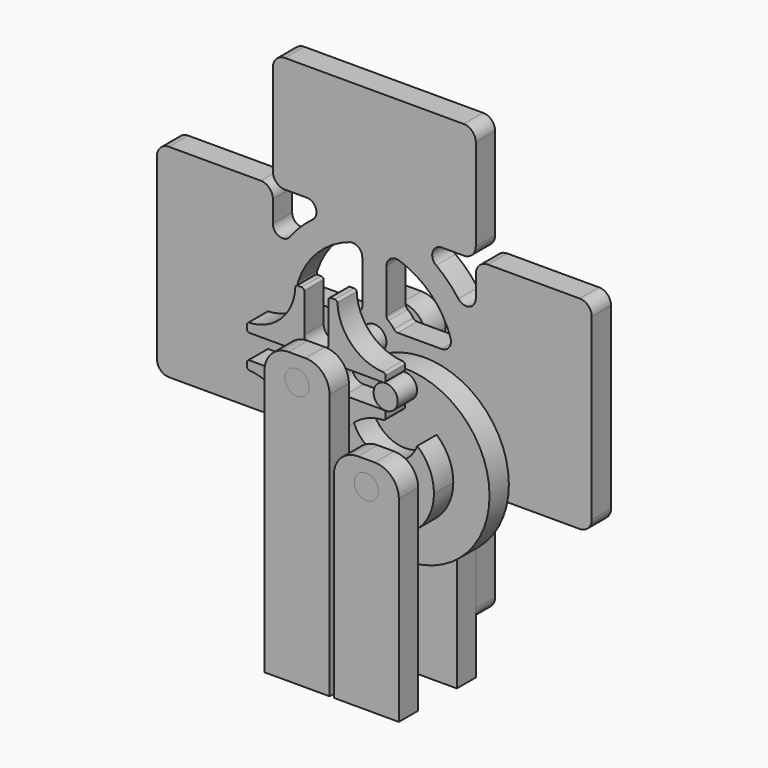
from build123d import *

# Parameters (mm, degrees)
F0_R          = 22.225
F0_R_2        = 3.175
F1_DEPTH      = 6.35
F2_DEPTH      = 6.35
F3_R          = 3.175
F4_DEPTH      = 6.35
F5_DEPTH      = 12.7
F5_DEPTH_BACK = 12.7
F6_DEPTH      = 12.7
F6_DEPTH_BACK = 25.4
F7_R          = 3.17499
F8_R          = 0.635
F9_W          = 17.0939071104
F9_H          = 57.9826636136
F9_R          = 3.175
F10_DEPTH     = 6.35
F9_H_2        = 76.2
F11_W         = 17.0939071104
F11_H         = 57.9826636136
F11_R         = 3.175
F12_DEPTH     = 6.35
F13_R         = 3.175
F13_W         = 11.8072872561
F13_H         = 12.7
F13_W_2       = 12.7
F13_H_2       = 11.8072872561
F14_DEPTH     = 6.35
F16_DEPTH     = 6.35
F17_R         = 2.54
F18_R         = 1.27
F19_W         = 17.0939071104
F19_H         = 76.2
F19_R         = 3.175
F20_DEPTH     = 6.35
F21_R         = 6.35
F21_2_R       = 6.35
F21_3_R       = 6.35
F21_4_R       = 6.35


# Not quite as in the source:
# - a fillet or chamfer is up to 0.001 mm smaller than in the source, because OpenCascade refuses the exact size
# - a feature names something its author has since deleted; it is built from what else it names


with BuildPart() as f1:
    # F0 (on Front) → F1 (new body)
    with BuildSketch(Plane.XZ):
        Circle(F0_R)
        with BuildLine():
            ThreePointArc((8.3277048309, 9.5885), (11.5553418676, 5.2691625828), (12.7, 0))
            ThreePointArc((12.7, 0), (-5.2691625828, -11.5553418676), (-8.3277048309, 9.5885))
            ThreePointArc((-8.3277048309, 9.5885), (0, 12.7), (8.3277048309, 9.5885))
        make_face(mode=Mode.SUBTRACT)
        with Locations((0, 18.2173363864)):
            Circle(F0_R_2, mode=Mode.SUBTRACT)
        with Locations((0, 18.2173363864)):
            Circle(F0_R_2)
        with BuildLine():
            ThreePointArc((-8.3277048309, 9.5885), (0, 3.81), (8.3277048309, 9.5885))
            ThreePointArc((8.3277048309, 9.5885), (0, 12.7), (-8.3277048309, 9.5885))
        make_face()
        with BuildLine():
            ThreePointArc((-8.3277048309, 9.5885), (-5.2691625828, -11.5553418676), (12.7, 0))
            ThreePointArc((12.7, 0), (11.5553418676, 5.2691625828), (8.3277048309, 9.5885))
            ThreePointArc((8.3277048309, 9.5885), (0, 3.81), (-8.3277048309, 9.5885))
        make_face()
        Circle(F0_R_2, mode=Mode.SUBTRACT)
    extrude(amount=-F1_DEPTH)

    # F0 (on Front) → F2 (join)
    with BuildSketch(Plane.XZ):
        with Locations((0, 18.2173363864)):
            Circle(F0_R_2)
        with BuildLine():
            ThreePointArc((-8.3277048309, 9.5885), (-5.2691625828, -11.5553418676), (12.7, 0))
            ThreePointArc((12.7, 0), (11.5553418676, 5.2691625828), (8.3277048309, 9.5885))
            ThreePointArc((8.3277048309, 9.5885), (0, 3.81), (-8.3277048309, 9.5885))
        make_face()
        Circle(F0_R_2, mode=Mode.SUBTRACT)
    extrude(amount=F2_DEPTH)


with BuildPart() as f4:
    # F3 (on face) → F4 (new body)
    with BuildSketch(Plane.XZ):
        with BuildLine():
            Line((-15.0423363864, 0), (-12.7, 0))
            ThreePointArc((-12.7, 0), (-11.5553418676, 5.2691625828), (-8.3277048309, 9.5885))
            ThreePointArc((-8.3277048309, 9.5885), (-4.445, 11.8967211869), (0, 12.7))
            Line((0, 12.7), (0, 15.0423363864))
            Line((0, 15.0423363864), (-13.97, 15.0423363864))
            Line((-13.97, 15.0423363864), (-13.97, 17.2855351378))
            ThreePointArc((-13.97, 17.2855351378), (-15.7154482119, 15.7154482119), (-17.2855351378, 13.97))
            Line((-17.2855351378, 13.97), (-15.0423363864, 13.97))
            Line((-15.0423363864, 13.97), (-15.0423363864, 0))
        make_face()
        with BuildLine():
            Line((-23.7346727729, 0), (-22.225, 0))
            ThreePointArc((-22.225, 0), (-22.0158499857, 3.0418702151), (-21.3923363864, 6.0264889388))
            Line((-21.3923363864, 6.0264889388), (-21.3923363864, 13.97))
            Line((-21.3923363864, 13.97), (-17.2855351378, 13.97))
            ThreePointArc((-17.2855351378, 13.97), (-15.7154482119, 15.7154482119), (-13.97, 17.2855351378))
            Line((-13.97, 17.2855351378), (-13.97, 21.3923363864))
            Line((-13.97, 21.3923363864), (-6.0264889388, 21.3923363864))
            ThreePointArc((-6.0264889388, 21.3923363864), (-3.0418702151, 22.0158499857), (0, 22.225))
            Line((0, 22.225), (0, 23.7346727729))
            ThreePointArc((0, 23.7346727729), (-8.9802561211, 27.4544166518), (-12.7, 36.4346727729))
            Line((-12.7, 36.4346727729), (-15.0423363864, 36.4346727729))
            Line((-15.0423363864, 36.4346727729), (-15.0423363864, 22.4646727729))
            Line((-15.0423363864, 22.4646727729), (-21.3923363864, 22.4646727729))
            Line((-21.3923363864, 22.4646727729), (-21.3923363864, 36.4346727729))
            Line((-21.3923363864, 36.4346727729), (-23.7346727729, 36.4346727729))
            ThreePointArc((-23.7346727729, 36.4346727729), (-27.4544166518, 27.4544166518), (-36.4346727729, 23.7346727729))
            Line((-36.4346727729, 23.7346727729), (-36.4346727729, 21.3923363864))
            Line((-36.4346727729, 21.3923363864), (-22.4646727729, 21.3923363864))
            Line((-22.4646727729, 21.3923363864), (-22.4646727729, 15.0423363864))
            Line((-22.4646727729, 15.0423363864), (-36.4346727729, 15.0423363864))
            Line((-36.4346727729, 15.0423363864), (-36.4346727729, 12.7))
            ThreePointArc((-36.4346727729, 12.7), (-27.4544166518, 8.9802561211), (-23.7346727729, 0))
        make_face()
        with Locations((-18.2173363864, 18.2173363864)):
            Circle(F3_R, mode=Mode.SUBTRACT)
        with BuildLine():
            Line((-6.0264889388, 21.3923363864), (0, 21.3923363864))
            Line((0, 21.3923363864), (0, 22.225))
            ThreePointArc((0, 22.225), (-3.0418702151, 22.0158499857), (-6.0264889388, 21.3923363864))
        make_face()
        with BuildLine():
            Line((-22.225, 0), (-21.3923363864, 0))
            Line((-21.3923363864, 0), (-21.3923363864, 6.0264889388))
            ThreePointArc((-21.3923363864, 6.0264889388), (-22.0158499857, 3.0418702151), (-22.225, 0))
        make_face()
    extrude(amount=F4_DEPTH)

    # F7 (radius 3.175 in the source; OpenCascade refuses exactly that, so slightly less here)
    f7_edges = [f4.edges().sort_by_distance(p)[0] for p in [
        (-15.042336, -3.175, 22.464673),
        (-21.392336, -3.175, 22.464673),
        (-13.97, -3.175, 21.392336),
        (-13.97, -3.175, 15.042336),
        (-15.042336, -3.175, 13.97),
        (-21.392336, -3.175, 13.97),
        (-22.464673, -3.175, 15.042336),
        (-22.464673, -3.175, 21.392336),
    ]]
    fillet(f7_edges, radius=F7_R)

    # F8
    f8_edges = [f4.edges().sort_by_distance(p)[0] for p in [
        (-12.7, -3.175, 36.434673),
        (-15.042336, -3.175, 36.434673),
        (-21.392336, -3.175, 36.434673),
        (-23.734673, -3.175, 36.434673),
        (-36.434673, -3.175, 23.734673),
        (0, -3.175, 23.734673),
        (0, -3.175, 21.392336),
        (0, -3.175, 12.7),
        (-36.434673, -3.175, 15.042336),
        (-21.392336, -3.175, 0),
        (-36.434673, -3.175, 21.392336),
        (-36.434673, -3.175, 12.7),
        (-23.734673, -3.175, 0),
        (-15.042336, -3.175, 0),
        (-12.7, -3.175, 0),
        (0, -3.175, 15.042336),
    ]]
    fillet(f8_edges, radius=F8_R)


with BuildPart() as f5:
    # F0 (on Front) → F5 (new body, two sides)
    with BuildSketch(Plane.XZ) as f5_sk:
        Circle(F0_R_2)
    extrude(amount=F5_DEPTH)
    extrude(f5_sk.sketch, amount=-F5_DEPTH_BACK)


with BuildPart() as f6:
    # F3 (on face) → F6 (new body, two sides)
    with BuildSketch(Plane.XZ) as f6_sk:
        with Locations((-18.2173363864, 18.2173363864)):
            Circle(F3_R)
    extrude(amount=F6_DEPTH)
    extrude(f6_sk.sketch, amount=-F6_DEPTH_BACK)


with BuildPart() as f10:
    # F9 (on face) → F10 (new body)
    with BuildSketch(Plane.XZ.offset(6.35)):
        with Locations((0, -22.6413318068)):
            Rectangle(F9_W, F9_H)
        Circle(F9_R, mode=Mode.SUBTRACT)
    extrude(amount=F10_DEPTH)

    # F21
    f21_edges = [f10.edges().sort_by_distance(p)[0] for p in [
        (8.546954, -9.525, 6.35),
        (-8.546954, -9.525, 6.35),
    ]]
    fillet(f21_edges, radius=F21_R)


with BuildPart() as f10b:
    # F9 (on face) → F10, piece 2 (new body)
    with BuildSketch(Plane.XZ.offset(6.35)):
        with Locations((-18.2173363864, -13.5326636136)):
            Rectangle(F9_W, F9_H_2)
        with Locations((-18.2173363864, 18.2173363864)):
            Circle(F9_R, mode=Mode.SUBTRACT)
    extrude(amount=F10_DEPTH)

    # F21#3
    f21_3_edges = [f10b.edges().sort_by_distance(p)[0] for p in [
        (-9.670383, -9.525, 24.567336),
        (-26.76429, -9.525, 24.567336),
    ]]
    fillet(f21_3_edges, radius=F21_3_R)


with BuildPart() as f12:
    # F11 (on face) → F12 (new body)
    with BuildSketch(Plane(origin=(0, 6.35, 0), x_dir=(-1, 0, 0), z_dir=(0, 1, 0))):
        with Locations((0, -22.6413318068)):
            Rectangle(F11_W, F11_H)
        Circle(F11_R, mode=Mode.SUBTRACT)
    extrude(amount=F12_DEPTH)

    # F21#2
    f21_2_edges = [f12.edges().sort_by_distance(p)[0] for p in [
        (8.546954, 9.525, 6.35),
        (-8.546954, 9.525, 6.35),
    ]]
    fillet(f21_2_edges, radius=F21_2_R)


with BuildPart() as f14:
    # F13 (on face) → F14 (new body)
    with BuildSketch(Plane(origin=(0, 12.7, 0), x_dir=(-1, 0, 0), z_dir=(0, 1, 0))):
        with BuildLine():
            ThreePointArc((44.8873363864, 11.8673363864), (45.4458475553, 15.0205286778), (45.6328684805, 18.2173363864))
            ThreePointArc((45.6328684805, 18.2173363864), (45.4458475553, 21.4141440951), (44.8873363864, 24.5673363864))
            Line((44.8873363864, 24.5673363864), (44.8873363864, 11.8673363864))
        make_face()
        with BuildLine():
            ThreePointArc((44.8873363864, 24.5673363864), (45.4458475553, 21.4141440951), (45.6328684805, 18.2173363864))
            ThreePointArc((45.6328684805, 18.2173363864), (45.4458475553, 15.0205286778), (44.8873363864, 11.8673363864))
            Line((44.8873363864, 11.8673363864), (44.8873363864, -5.2776636136))
            ThreePointArc((44.8873363864, -5.2776636136), (45.8172723562, -7.5227276438), (48.0623363864, -8.4526636136))
            Line((48.0623363864, -8.4526636136), (72.1923363864, -8.4526636136))
            ThreePointArc((72.1923363864, -8.4526636136), (74.4374004167, -7.5227276438), (75.3673363864, -5.2776636136))
            Line((75.3673363864, -5.2776636136), (75.3673363864, 41.7123363864))
            ThreePointArc((75.3673363864, 41.7123363864), (74.4374004167, 43.9574004167), (72.1923363864, 44.8873363864))
            Line((72.1923363864, 44.8873363864), (48.0623363864, 44.8873363864))
            ThreePointArc((48.0623363864, 44.8873363864), (45.8172723562, 43.9574004167), (44.8873363864, 41.7123363864))
            Line((44.8873363864, 41.7123363864), (44.8873363864, 24.5673363864))
        make_face()
        with BuildLine():
            Line((33.0800491303, 24.5673363864), (44.8873363864, 24.5673363864))
            ThreePointArc((44.8873363864, 24.5673363864), (37.60304504, 37.60304504), (24.5673363864, 44.8873363864))
            Line((24.5673363864, 44.8873363864), (24.5673363864, 33.0800491303))
            Line((24.5673363864, 33.0800491303), (11.8673363864, 33.0800491303))
            Line((11.8673363864, 33.0800491303), (11.8673363864, 44.8873363864))
            ThreePointArc((11.8673363864, 44.8873363864), (-1.1683722671, 37.60304504), (-8.4526636136, 24.5673363864))
            Line((-8.4526636136, 24.5673363864), (3.3546236426, 24.5673363864))
            Line((3.3546236426, 24.5673363864), (3.3546236426, 11.8673363864))
            Line((3.3546236426, 11.8673363864), (-8.4526636136, 11.8673363864))
            ThreePointArc((-8.4526636136, 11.8673363864), (-1.1683722671, -1.1683722671), (11.8673363864, -8.4526636136))
            Line((11.8673363864, -8.4526636136), (11.8673363864, 3.3546236426))
            Line((11.8673363864, 3.3546236426), (24.5673363864, 3.3546236426))
            Line((24.5673363864, 3.3546236426), (24.5673363864, -8.4526636136))
            ThreePointArc((24.5673363864, -8.4526636136), (37.60304504, -1.1683722671), (44.8873363864, 11.8673363864))
            Line((44.8873363864, 11.8673363864), (33.0800491303, 11.8673363864))
            Line((33.0800491303, 11.8673363864), (33.0800491303, 24.5673363864))
        make_face()
        with Locations((18.2173363864, 18.2173363864)):
            Circle(F13_R, mode=Mode.SUBTRACT)
        with Locations((38.9836927584, 18.2173363864)):
            Rectangle(F13_W, F13_H)
        with BuildLine():
            Line((11.8673363864, 44.8873363864), (24.5673363864, 44.8873363864))
            ThreePointArc((24.5673363864, 44.8873363864), (18.2173363864, 45.6328684805), (11.8673363864, 44.8873363864))
        make_face()
        with Locations((18.2173363864, 38.9836927584)):
            Rectangle(F13_W_2, F13_H_2)
        with BuildLine():
            ThreePointArc((11.8673363864, 44.8873363864), (18.2173363864, 45.6328684805), (24.5673363864, 44.8873363864))
            Line((24.5673363864, 44.8873363864), (41.7123363864, 44.8873363864))
            ThreePointArc((41.7123363864, 44.8873363864), (43.9574004167, 45.8172723562), (44.8873363864, 48.0623363864))
            Line((44.8873363864, 48.0623363864), (44.8873363864, 72.1923363864))
            ThreePointArc((44.8873363864, 72.1923363864), (43.9574004167, 74.4374004167), (41.7123363864, 75.3673363864))
            Line((41.7123363864, 75.3673363864), (-5.2776636136, 75.3673363864))
            ThreePointArc((-5.2776636136, 75.3673363864), (-7.5227276438, 74.4374004167), (-8.4526636136, 72.1923363864))
            Line((-8.4526636136, 72.1923363864), (-8.4526636136, 48.0623363864))
            ThreePointArc((-8.4526636136, 48.0623363864), (-7.5227276438, 45.8172723562), (-5.2776636136, 44.8873363864))
            Line((-5.2776636136, 44.8873363864), (11.8673363864, 44.8873363864))
        make_face()
        with BuildLine():
            Line((41.7123363864, -8.4526636136), (24.5673363864, -8.4526636136))
            ThreePointArc((24.5673363864, -8.4526636136), (18.2173363864, -9.1981957076), (11.8673363864, -8.4526636136))
            Line((11.8673363864, -8.4526636136), (-5.2776636136, -8.4526636136))
            ThreePointArc((-5.2776636136, -8.4526636136), (-7.5227276438, -9.3825995833), (-8.4526636136, -11.6276636136))
            Line((-8.4526636136, -11.6276636136), (-8.4526636136, -35.7576636136))
            ThreePointArc((-8.4526636136, -35.7576636136), (-7.5227276438, -38.0027276438), (-5.2776636136, -38.9326636136))
            Line((-5.2776636136, -38.9326636136), (41.7123363864, -38.9326636136))
            ThreePointArc((41.7123363864, -38.9326636136), (43.9574004167, -38.0027276438), (44.8873363864, -35.7576636136))
            Line((44.8873363864, -35.7576636136), (44.8873363864, -11.6276636136))
            ThreePointArc((44.8873363864, -11.6276636136), (43.9574004167, -9.3825995833), (41.7123363864, -8.4526636136))
        make_face()
        with BuildLine():
            ThreePointArc((11.8673363864, -8.4526636136), (18.2173363864, -9.1981957076), (24.5673363864, -8.4526636136))
            Line((24.5673363864, -8.4526636136), (11.8673363864, -8.4526636136))
        make_face()
        with Locations((18.2173363864, -2.5490199855)):
            Rectangle(F13_W_2, F13_H_2)
        with BuildLine():
            Line((-8.4526636136, 11.8673363864), (-8.4526636136, 24.5673363864))
            ThreePointArc((-8.4526636136, 24.5673363864), (-9.1981957076, 18.2173363864), (-8.4526636136, 11.8673363864))
        make_face()
        with Locations((-2.5490199855, 18.2173363864)):
            Rectangle(F13_W, F13_H)
        with BuildLine():
            ThreePointArc((-8.4526636136, 11.8673363864), (-9.1981957076, 18.2173363864), (-8.4526636136, 24.5673363864))
            Line((-8.4526636136, 24.5673363864), (-8.4526636136, 41.7123363864))
            ThreePointArc((-8.4526636136, 41.7123363864), (-9.3825995833, 43.9574004167), (-11.6276636136, 44.8873363864))
            Line((-11.6276636136, 44.8873363864), (-35.7576636136, 44.8873363864))
            ThreePointArc((-35.7576636136, 44.8873363864), (-38.0027276438, 43.9574004167), (-38.9326636136, 41.7123363864))
            Line((-38.9326636136, 41.7123363864), (-38.9326636136, -5.2776636136))
            ThreePointArc((-38.9326636136, -5.2776636136), (-38.0027276438, -7.5227276438), (-35.7576636136, -8.4526636136))
            Line((-35.7576636136, -8.4526636136), (-11.6276636136, -8.4526636136))
            ThreePointArc((-11.6276636136, -8.4526636136), (-9.3825995833, -7.5227276438), (-8.4526636136, -5.2776636136))
            Line((-8.4526636136, -5.2776636136), (-8.4526636136, 11.8673363864))
        make_face()
    extrude(amount=F14_DEPTH)

    # F15 (on face) → F16 (cut, through all)
    with BuildSketch(Plane(origin=(0, 19.05, 0), x_dir=(-1, 0, 0), z_dir=(0, 1, 0))):
        with BuildLine():
            ThreePointArc((39.0422257596, 21.3923363864), (33.1129169794, 33.1129169794), (21.3923363864, 39.0422257596))
            Line((21.3923363864, 39.0422257596), (21.3923363864, 23.7165977005))
            ThreePointArc((21.3923363864, 23.7165977005), (22.707464447, 22.707464447), (23.7165977005, 21.3923363864))
            Line((23.7165977005, 21.3923363864), (39.0422257596, 21.3923363864))
        make_face()
        with BuildLine():
            Line((39.0422257596, 15.0423363864), (23.7165977005, 15.0423363864))
            ThreePointArc((23.7165977005, 15.0423363864), (22.707464447, 13.7272083259), (21.3923363864, 12.7180750724))
            Line((21.3923363864, 12.7180750724), (21.3923363864, -2.6075529867))
            ThreePointArc((21.3923363864, -2.6075529867), (33.1129169794, 3.3217557934), (39.0422257596, 15.0423363864))
        make_face()
        with BuildLine():
            ThreePointArc((15.0423363864, 12.7180750724), (13.7272083259, 13.7272083259), (12.7180750724, 15.0423363864))
            Line((12.7180750724, 15.0423363864), (-2.6075529867, 15.0423363864))
            ThreePointArc((-2.6075529867, 15.0423363864), (3.3217557934, 3.3217557934), (15.0423363864, -2.6075529867))
            Line((15.0423363864, -2.6075529867), (15.0423363864, 12.7180750724))
        make_face()
        with BuildLine():
            ThreePointArc((12.7180750724, 21.3923363864), (13.7272083259, 22.707464447), (15.0423363864, 23.7165977005))
            Line((15.0423363864, 23.7165977005), (15.0423363864, 39.0422257596))
            ThreePointArc((15.0423363864, 39.0422257596), (3.3217557934, 33.1129169794), (-2.6075529867, 21.3923363864))
            Line((-2.6075529867, 21.3923363864), (12.7180750724, 21.3923363864))
        make_face()
    extrude(amount=-F16_DEPTH, mode=Mode.SUBTRACT)

    # F17
    f17_edges = [f14.edges().sort_by_distance(p)[0] for p in [
        (-11.867336, 15.875, 44.887336),
        (-24.567336, 15.875, 44.887336),
        (-44.887336, 15.875, 24.567336),
        (8.452664, 15.875, 24.567336),
        (8.452664, 15.875, 11.867336),
        (-44.887336, 15.875, 11.867336),
        (-24.567336, 15.875, -8.452664),
        (-11.867336, 15.875, -8.452664),
        (-15.042336, 15.875, 39.042226),
        (2.607553, 15.875, 21.392336),
        (-21.392336, 15.875, 39.042226),
        (-39.042226, 15.875, 21.392336),
        (2.607553, 15.875, 15.042336),
        (-15.042336, 15.875, -2.607553),
        (-21.392336, 15.875, -2.607553),
    ]]
    fillet(f17_edges, radius=F17_R)

    # F18
    f18_edges = [f14.edges().sort_by_distance(p)[0] for p in [
        (-15.042336, 15.875, 23.716598),
        (-12.718075, 15.875, 21.392336),
        (-21.392336, 15.875, 23.716598),
        (-23.716598, 15.875, 21.392336),
        (-23.716598, 15.875, 15.042336),
        (-21.392336, 15.875, 12.718075),
        (-12.718075, 15.875, 15.042336),
        (-15.042336, 15.875, 12.718075),
    ]]
    fillet(f18_edges, radius=F18_R)


with BuildPart() as f20:
    # F19 (on face) → F20 (new body)
    with BuildSketch(Plane(origin=(0, 19.05, 0), x_dir=(-1, 0, 0), z_dir=(0, 1, 0))):
        with Locations((18.2173363864, -13.5326636136)):
            Rectangle(F19_W, F19_H)
        with Locations((18.2173363864, 18.2173363864)):
            Circle(F19_R, mode=Mode.SUBTRACT)
    extrude(amount=F20_DEPTH)

    # F21#4
    f21_4_edges = [f20.edges().sort_by_distance(p)[0] for p in [
        (-9.670383, 22.225, 24.567336),
        (-26.76429, 22.225, 24.567336),
    ]]
    fillet(f21_4_edges, radius=F21_4_R)


solid = Compound([f1.part, f4.part, f5.part, f6.part, f10.part, f10b.part, f12.part, f14.part, f20.part])
